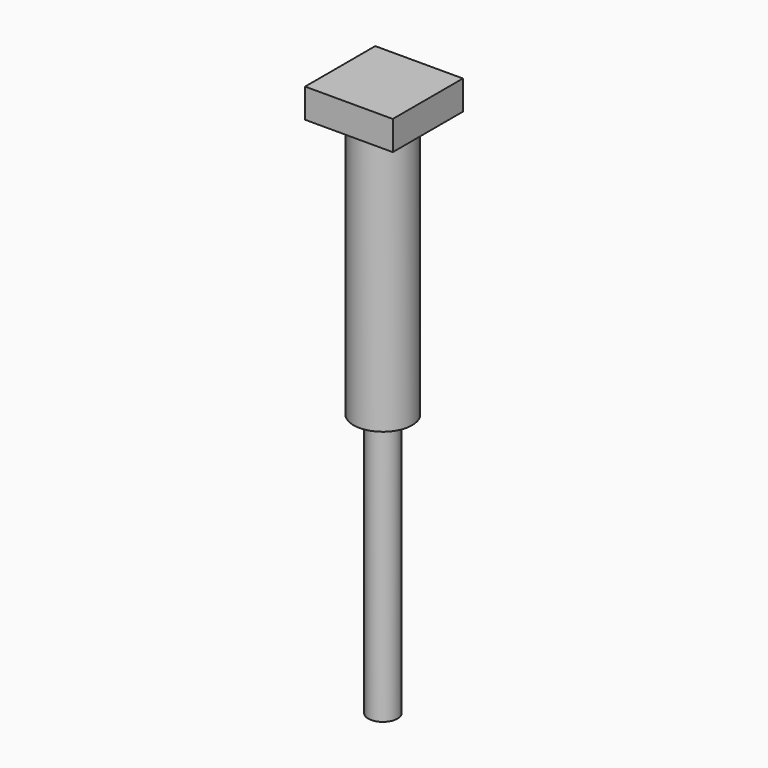
from build123d import *

# Parameters (mm, degrees)
F0_W     = 7.62
F0_H     = 7.62
F1_DEPTH = 2.54
F2_R     = 2.54
F2_R_2   = 1.27
F3_DEPTH = 22.86
F4_DEPTH = 22.86
F5_DEPTH = 45.72
F6_R     = 0.254
F7_DEPTH = 2.54


# Not quite as in the source:
# - a feature names something its author has since deleted; it is built from what else it names


with BuildPart() as f1:
    # F0 (on Top) → F1 (new body)
    with BuildSketch(Plane.XY):
        with Locations((-38.7955456972, -21.8359371471)):
            Rectangle(F0_W, F0_H)
    extrude(amount=F1_DEPTH)

    # F2 (on face) → F3 (join)
    with BuildSketch(Plane(origin=(0, 0, 0), x_dir=(1, 0, 0), z_dir=(0, 0, -1))):
        with Locations((-38.854431361, 21.8882076442)):
            Circle(F2_R)
        with Locations((-38.854431361, 21.8882076442)):
            Circle(F2_R_2, mode=Mode.SUBTRACT)
    extrude(amount=F3_DEPTH)

    # F4 (add): a face of the model
    f4_faces = [f1.faces().sort_by_distance(p)[0] for p in [
        (-38.854431361, -21.8882076442, 0),
    ]]
    extrude(f4_faces, amount=F4_DEPTH)

    # F2 (on face) → F5 (join)
    with BuildSketch(Plane(origin=(0, 0, 0), x_dir=(1, 0, 0), z_dir=(0, 0, -1))):
        with Locations((-38.854431361, 21.8882076442)):
            Circle(F2_R_2)
    extrude(amount=F5_DEPTH)

    # F6 (on face) → F7 (cut)
    with BuildSketch(Plane(origin=(0, 0, -45.72), x_dir=(1, 0, 0), z_dir=(0, 0, -1))):
        with Locations((-38.854431361, 21.8882076442)):
            Circle(F6_R)
    extrude(amount=-F7_DEPTH, mode=Mode.SUBTRACT)


solid = f1.part
